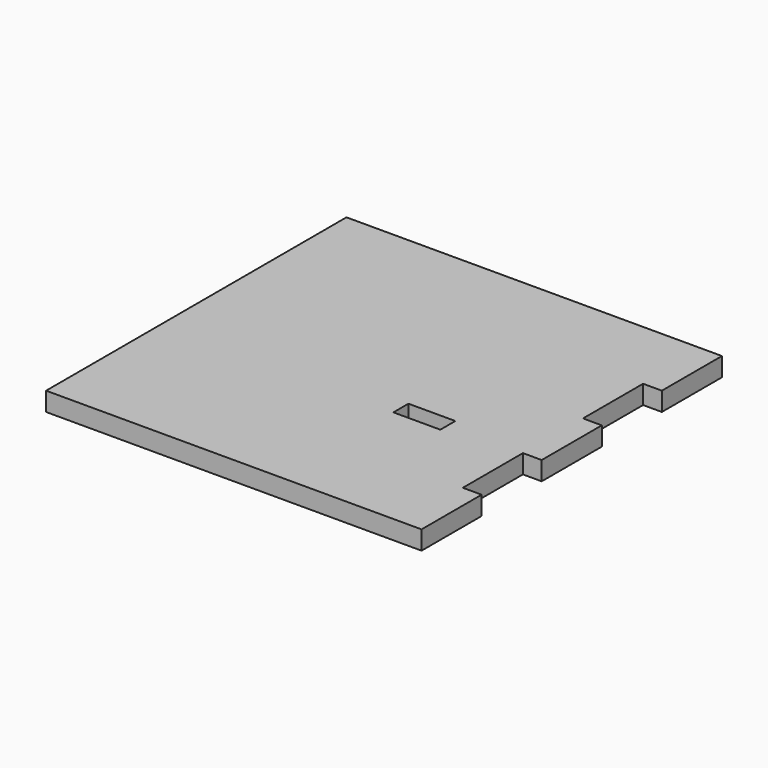
from build123d import *

# Parameters (mm, degrees)
F0_DEPTH = 2
F1_W     = 5
F1_H     = 2
F3_DEPTH = 2


# Not quite as in the source:
# - a feature names something its author has since deleted; it is built from what else it names


with BuildPart() as f0:
    # F2 (on Top) → F0 (new body)
    with BuildSketch(Plane.XY):
        Polygon((2, 40), (2, 0), (42, 0), (42, 8), (40, 8), (40, 16), (42, 16), (42, 24), (40, 24), (40, 32), (42, 32), (42, 40), align=None)
    extrude(amount=F0_DEPTH)

    # F1 (on Top) → F3 (cut)
    with BuildSketch(Plane.XY):
        with Locations((29.5, 16)):
            Rectangle(F1_W, F1_H)
    extrude(amount=F3_DEPTH, mode=Mode.SUBTRACT)


solid = f0.part
